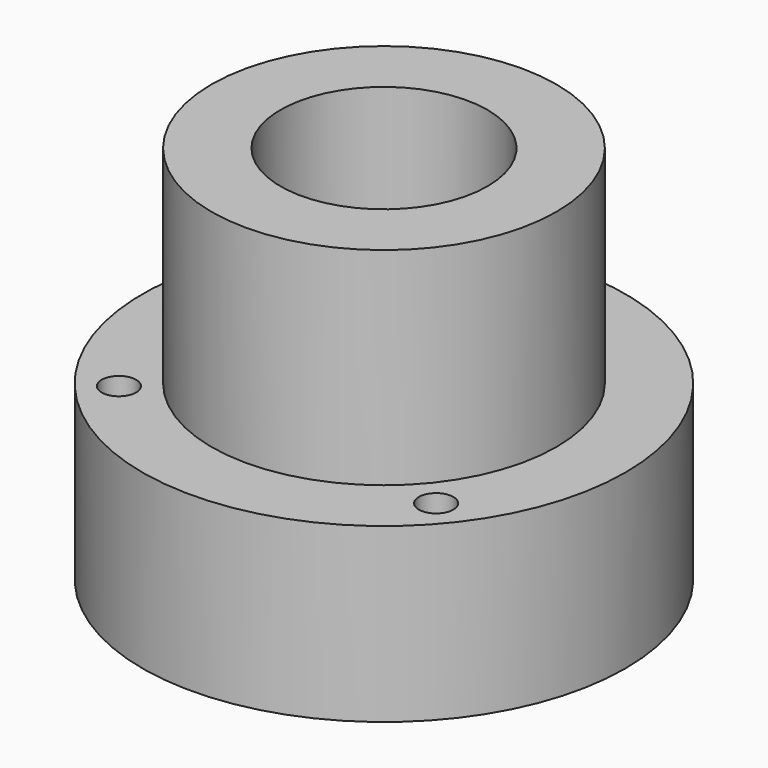
from build123d import *

# Parameters (mm, degrees)
F0_R     = 35
F0_R_2   = 2.5
F0_R_3   = 25
F1_DEPTH = 25
F0_R_4   = 15
F2_DEPTH = 55


# Not quite as in the source:
# - the program builds the solid bodies; features that only make, move or delete a surface that nothing else refers to are left out


with BuildPart() as f1:
    # F0 (on Top) → F1 (new body)
    with BuildSketch(Plane.XY):
        Circle(F0_R)
        with Locations((-22.9813332936, -19.2836282906)):
            Circle(F0_R_2, mode=Mode.SUBTRACT)
        with Locations((22.9813332936, -19.2836282906)):
            Circle(F0_R_2, mode=Mode.SUBTRACT)
        Circle(F0_R_3, mode=Mode.SUBTRACT)
        with Locations((0, 30)):
            Circle(F0_R_2, mode=Mode.SUBTRACT)
    extrude(amount=F1_DEPTH)

    # F0 (on Top) → F2 (join)
    with BuildSketch(Plane.XY):
        Circle(F0_R_3)
        Circle(F0_R_4, mode=Mode.SUBTRACT)
    extrude(amount=F2_DEPTH)


solid = f1.part
